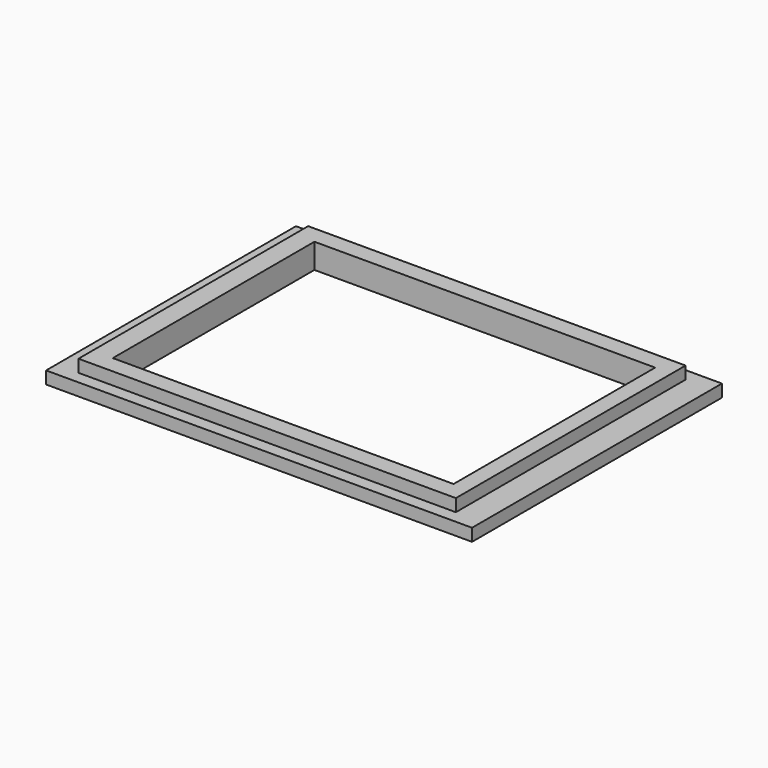
from build123d import *

# Parameters (mm, degrees)
F0_W     = 381
F0_H     = 279.4
F0_W_2   = 304.8
F0_H_2   = 225.425
F1_DEPTH = 11.1125
F2_W     = 337.566
F2_H     = 256.794
F2_W_2   = 304.8
F2_H_2   = 225.425
F3_DEPTH = 11.1125


# Not quite as in the source:
# - a length typed as a fraction of an inch, garbled in the dataset ("3 / 203.2 mm" for 3/8 in), is restored


with BuildPart() as f1:
    # F0 (on Top) → F1 (new body)
    with BuildSketch(Plane.XY):
        with Locations((2.4245437235, -40.6000330182)):
            Rectangle(F0_W, F0_H)
        with Locations((2.4245437235, -40.6000330182)):
            Rectangle(F0_W_2, F0_H_2, mode=Mode.SUBTRACT)
    extrude(amount=F1_DEPTH)

    # F2 (on face) → F3 (join)
    with BuildSketch(Plane.XY.offset(11.1125)):
        with Locations((0.6465390325, -40.6000330182)):
            Rectangle(F2_W, F2_H)
        with Locations((2.4245437235, -40.6000330182)):
            Rectangle(F2_W_2, F2_H_2, mode=Mode.SUBTRACT)
    extrude(amount=F3_DEPTH)


solid = f1.part
